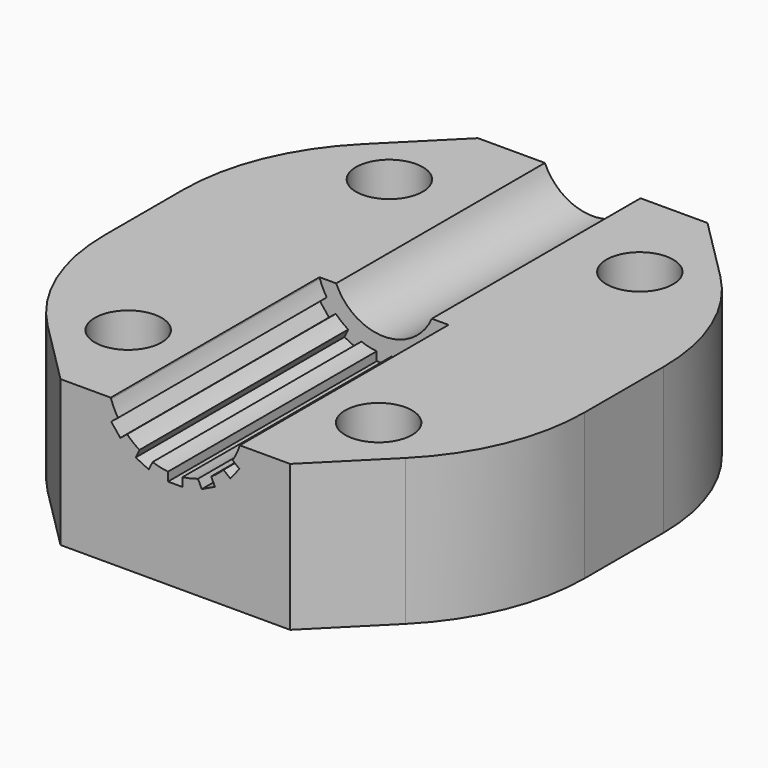
from build123d import *

# Parameters (mm, degrees)
F0_W     = 23
F0_H     = 25
F1_DEPTH = 7
F3_DEPTH = 25.001
F4_DEPTH = 12.5
F5_SIZE  = 6
F6_R     = 10
F7_R     = 1.6
F8_DEPTH = 25


with BuildPart() as f1:
    # F0 (on Top) → F1 (new body)
    with BuildSketch(Plane.XY):
        Rectangle(F0_W, F0_H)
    extrude(amount=F1_DEPTH)

    # F2 (on face) → F3 (cut, through all)
    with BuildSketch(Plane.XZ.offset(12.5)):
        with BuildLine():
            Line((0, 7), (-2.2912878475, 7))
            ThreePointArc((-2.2912878475, 7), (0, 5.5), (2.2912878475, 7))
            Line((2.2912878475, 7), (0, 7))
        make_face()
    extrude(amount=-F3_DEPTH, mode=Mode.SUBTRACT)

    # F2 (on face) → F4 (cut)
    with BuildSketch(Plane.XZ.offset(12.5)):
        with BuildLine():
            ThreePointArc((2.2912878475, 7), (0, 5.5), (-2.2912878475, 7))
            Line((-2.2912878475, 7), (-2.8084005449, 7))
            Line((-2.8084005449, 7), (-3.0722061624, 6.9397880893))
            ThreePointArc((-3.0722061624, 6.9397880893), (-2.9281488207, 6.5898778479), (-2.7443962613, 6.2590838157))
            Line((-2.7443962613, 6.2590838157), (-2.4464411557, 6.4966950836))
            Line((-2.4464411557, 6.4966950836), (-2.0099982944, 5.9494130458))
            Line((-2.0099982944, 5.9494130458), (-2.3079534, 5.711801778))
            ThreePointArc((-2.3079534, 5.711801778), (-2.026341856, 5.459047682), (-1.7172603691, 5.2407398048))
            Line((-1.7172603691, 5.2407398048), (-1.5519077603, 5.5840980352))
            Line((-1.5519077603, 5.5840980352), (-0.9212295527, 5.2803794178))
            Line((-0.9212295527, 5.2803794178), (-1.0865821616, 4.9370211875))
            ThreePointArc((-1.0865821616, 4.9370211875), (-0.7231930354, 4.8314842854), (-0.35, 4.7689011157))
            Line((-0.35, 4.7689011157), (-0.35, 5.15))
            Line((-0.35, 5.15), (0.35, 5.15))
            Line((0.35, 5.15), (0.35, 4.7689011157))
            ThreePointArc((0.35, 4.7689011157), (0.7231930354, 4.8314842854), (1.0865821616, 4.9370211875))
            Line((1.0865821616, 4.9370211875), (0.9212295527, 5.2803794178))
            Line((0.9212295527, 5.2803794178), (1.5519077603, 5.5840980352))
            Line((1.5519077603, 5.5840980352), (1.7172603691, 5.2407398048))
            ThreePointArc((1.7172603691, 5.2407398048), (2.026341856, 5.459047682), (2.3079534, 5.711801778))
            Line((2.3079534, 5.711801778), (2.0099982944, 5.9494130458))
            Line((2.0099982944, 5.9494130458), (2.4464411557, 6.4966950836))
            Line((2.4464411557, 6.4966950836), (2.7443962613, 6.2590838157))
            ThreePointArc((2.7443962613, 6.2590838157), (2.9281488207, 6.5898778479), (3.0722061624, 6.9397880893))
            Line((3.0722061624, 6.9397880893), (2.8084005449, 7))
            Line((2.8084005449, 7), (2.2912878475, 7))
        make_face()
        with BuildLine():
            Line((3.0719063417, 5.9979032421), (2.7443962613, 6.2590838157))
            ThreePointArc((2.7443962613, 6.2590838157), (2.540952318, 5.973658144), (2.3079534, 5.711801778))
            Line((2.3079534, 5.711801778), (2.6354634804, 5.4506212044))
            Line((2.6354634804, 5.4506212044), (3.0719063417, 5.9979032421))
        make_face()
        with BuildLine():
            ThreePointArc((2.3079534, 5.711801778), (2.540952318, 5.973658144), (2.7443962613, 6.2590838157))
            Line((2.7443962613, 6.2590838157), (2.4464411557, 6.4966950836))
            Line((2.4464411557, 6.4966950836), (2.0099982944, 5.9494130458))
            Line((2.0099982944, 5.9494130458), (2.3079534, 5.711801778))
        make_face()
        with BuildLine():
            Line((1.8990147515, 4.8633229408), (1.7172603691, 5.2407398048))
            ThreePointArc((1.7172603691, 5.2407398048), (1.4101221521, 5.0718511793), (1.0865821616, 4.9370211875))
            Line((1.0865821616, 4.9370211875), (1.268336544, 4.5596043235))
            Line((1.268336544, 4.5596043235), (1.8990147515, 4.8633229408))
        make_face()
        with BuildLine():
            ThreePointArc((1.0865821616, 4.9370211875), (1.4101221521, 5.0718511793), (1.7172603691, 5.2407398048))
            Line((1.7172603691, 5.2407398048), (1.5519077603, 5.5840980352))
            Line((1.5519077603, 5.5840980352), (0.9212295527, 5.2803794178))
            Line((0.9212295527, 5.2803794178), (1.0865821616, 4.9370211875))
        make_face()
        with BuildLine():
            ThreePointArc((0.35, 4.7689011157), (0, 4.75), (-0.35, 4.7689011157))
            Line((-0.35, 4.7689011157), (-0.35, 4.35))
            Line((-0.35, 4.35), (0.35, 4.35))
            Line((0.35, 4.35), (0.35, 4.7689011157))
        make_face()
        with BuildLine():
            Line((-0.35, 5.15), (-0.35, 4.7689011157))
            ThreePointArc((-0.35, 4.7689011157), (0, 4.75), (0.35, 4.7689011157))
            Line((0.35, 4.7689011157), (0.35, 5.15))
            Line((0.35, 5.15), (-0.35, 5.15))
        make_face()
        with BuildLine():
            ThreePointArc((-1.0865821616, 4.9370211875), (-1.4101221521, 5.0718511793), (-1.7172603691, 5.2407398048))
            Line((-1.7172603691, 5.2407398048), (-1.8990147515, 4.8633229408))
            Line((-1.8990147515, 4.8633229408), (-1.268336544, 4.5596043235))
            Line((-1.268336544, 4.5596043235), (-1.0865821616, 4.9370211875))
        make_face()
        with BuildLine():
            Line((-1.5519077603, 5.5840980352), (-1.7172603691, 5.2407398048))
            ThreePointArc((-1.7172603691, 5.2407398048), (-1.4101221521, 5.0718511793), (-1.0865821616, 4.9370211875))
            Line((-1.0865821616, 4.9370211875), (-0.9212295527, 5.2803794178))
            Line((-0.9212295527, 5.2803794178), (-1.5519077603, 5.5840980352))
        make_face()
        with BuildLine():
            ThreePointArc((-2.3079534, 5.711801778), (-2.540952318, 5.973658144), (-2.7443962613, 6.2590838157))
            Line((-2.7443962613, 6.2590838157), (-3.0719063417, 5.9979032421))
            Line((-3.0719063417, 5.9979032421), (-2.6354634804, 5.4506212044))
            Line((-2.6354634804, 5.4506212044), (-2.3079534, 5.711801778))
        make_face()
        with BuildLine():
            Line((-2.4464411557, 6.4966950836), (-2.7443962613, 6.2590838157))
            ThreePointArc((-2.7443962613, 6.2590838157), (-2.540952318, 5.973658144), (-2.3079534, 5.711801778))
            Line((-2.3079534, 5.711801778), (-2.0099982944, 5.9494130458))
            Line((-2.0099982944, 5.9494130458), (-2.4464411557, 6.4966950836))
        make_face()
        with BuildLine():
            Line((3.0923292192, 7), (2.8084005449, 7))
            Line((2.8084005449, 7), (3.0722061624, 6.9397880893))
            ThreePointArc((3.0722061624, 6.9397880893), (3.0824147168, 6.969844908), (3.0923292192, 7))
        make_face()
        with BuildLine():
            Line((-3.0722061624, 6.9397880893), (-2.8084005449, 7))
            Line((-2.8084005449, 7), (-3.0923292192, 7))
            ThreePointArc((-3.0923292192, 7), (-3.0824147168, 6.969844908), (-3.0722061624, 6.9397880893))
        make_face()
    extrude(amount=-F4_DEPTH, mode=Mode.SUBTRACT)

    # F5
    f5_edges = [f1.edges().sort_by_distance(p)[0] for p in [
        (11.5, -12.5, 3.5),
        (-11.5, -12.5, 3.5),
        (11.5, 12.5, 3.5),
        (-11.5, 12.5, 3.5),
    ]]
    chamfer(f5_edges, length=F5_SIZE)

    # F6
    f6_edges = [f1.edges().sort_by_distance(p)[0] for p in [
        (11.5, 6.5, 3.5),
        (11.5, -6.5, 3.5),
        (-11.5, 6.5, 3.5),
        (-11.5, -6.5, 3.5),
    ]]
    fillet(f6_edges, radius=F6_R)

    # F7 (on face) → F8 (cut)
    with BuildSketch(Plane.XY.offset(7)):
        with Locations((6, -7.8212832158)):
            Circle(F7_R)
        with Locations((-6, -7.8212832158)):
            Circle(F7_R)
        with Locations((-6, 7.8212832158)):
            Circle(F7_R)
        with Locations((6, 7.8212832158)):
            Circle(F7_R)
    extrude(amount=-F8_DEPTH, mode=Mode.SUBTRACT)


solid = f1.part
